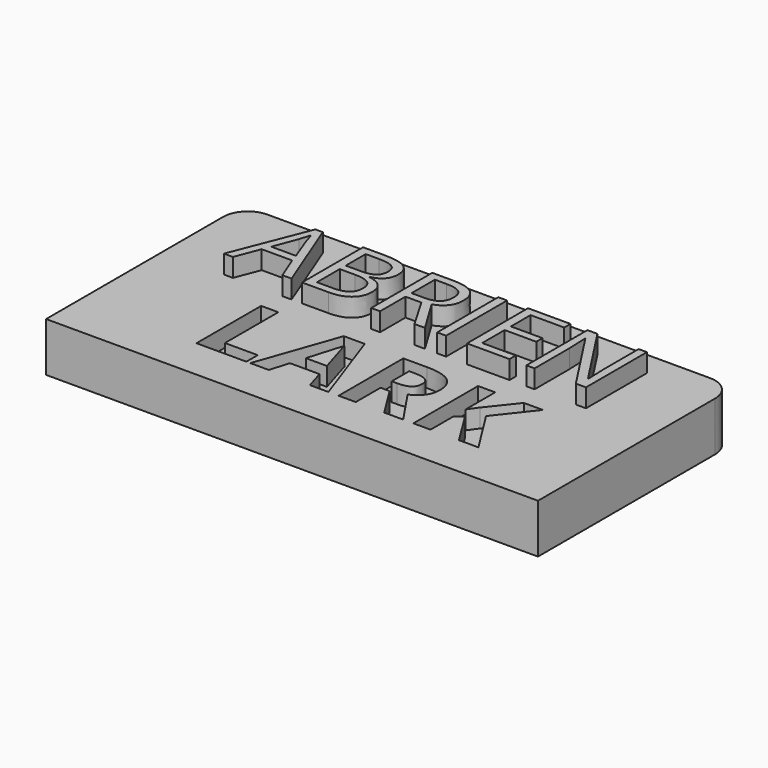
from build123d import *

# Parameters (mm, degrees)
F0_W         = 101.6
F0_H         = 50.8
F1_DEPTH     = 10.16
F3_TEXT_SIZE = 23.3928621229
F4_DEPTH     = 3.81
F2_TEXT_SIZE = 22.0589831735
F5_DEPTH     = 3.81
F6_R         = 5.08
F7_R         = 5.08


# Not quite as in the source:
# - Text() gives the source's letters only with a copy of the font that has no kerning and outlines rounded to 1/6400 em; it was checked with that copy


with BuildPart() as f1:
    # F0 (on Top) → F1 (new body)
    with BuildSketch(Plane.XY):
        Rectangle(F0_W, F0_H)
    extrude(amount=F1_DEPTH)

    # F3 (on face) → F4 (cut)
    with BuildSketch(Plane.XY.offset(10.16)):
        with Locations((-28.6868587136, -16.8428607285)):
            Text('LARK', F3_TEXT_SIZE, font='Open Sans', font_style=FontStyle.BOLD, text_align=(TextAlign.LEFT, TextAlign.BOTTOM))
    extrude(amount=-F4_DEPTH, mode=Mode.SUBTRACT)

    # F2 (on face) → F5 (join)
    with BuildSketch(Plane.XY.offset(10.16)):
        with Locations((-38.1, 4.649259704)):
            Text('ABRIEN', F2_TEXT_SIZE, font='Open Sans', text_align=(TextAlign.LEFT, TextAlign.BOTTOM))
    extrude(amount=F5_DEPTH)

    # F6
    f6_edges = [f1.edges().sort_by_distance(p)[0] for p in [
        (-50.8, 25.4, 5.08),
    ]]
    fillet(f6_edges, radius=F6_R)

    # F7
    f7_edges = [f1.edges().sort_by_distance(p)[0] for p in [
        (50.8, 25.4, 5.08),
    ]]
    fillet(f7_edges, radius=F7_R)


solid = f1.part
